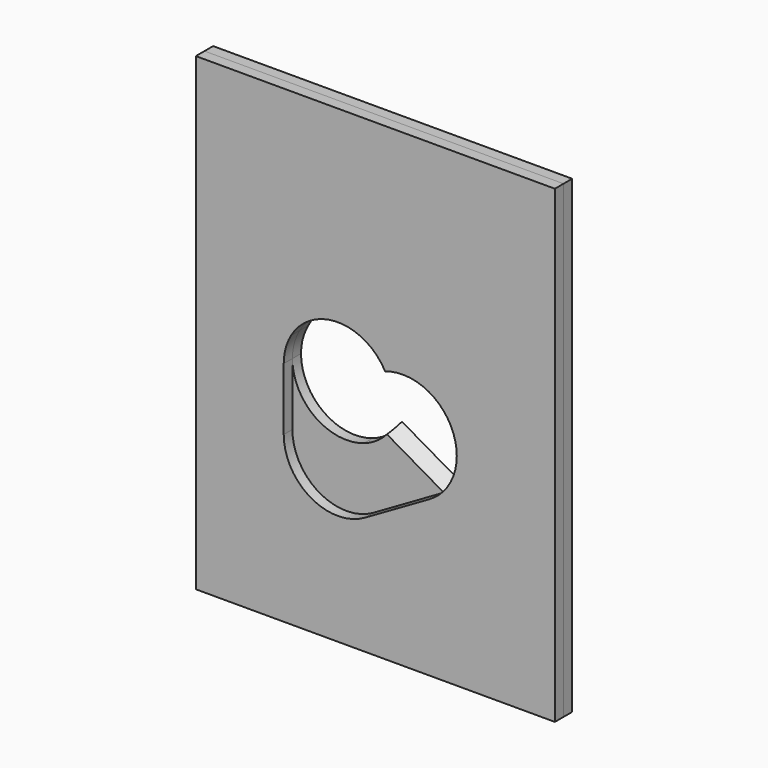
from build123d import *

# Parameters (mm, degrees)
F0_W     = 332.0041149855
F0_H     = 434.023141861
F1_DEPTH = 10
F2_DEPTH = 10
F3_SIZE  = 9.99999


# Not quite as in the source:
# - a fillet or chamfer is up to 0.001 mm smaller than in the source, because OpenCascade refuses the exact size


with BuildPart() as f1:
    # F0 (on Front) → F1 (new body)
    with BuildSketch(Plane.XZ):
        with Locations((34.709520638, 6.8919658661)):
            Rectangle(F0_W, F0_H)
        with BuildLine():
            ThreePointArc((-50, 0), (-48.2962913145, 12.9409522551), (-43.3012701892, 25))
            Line((-43.3012701892, 25), (16.6987298108, 128.9230484541))
            ThreePointArc((16.6987298108, 128.9230484541), (72.9409522551, 152.2193397686), (110, 103.9230484541))
            Line((110, 103.9230484541), (110, -23.0940107676))
            Line((110, -23.0940107676), (110, -63.5085296109))
            Line((110, -63.5085296109), (97.4264068712, -56.2491622333))
            ThreePointArc((97.4264068712, -56.2491622333), (91.6227766017, -61.8238442297), (85, -66.3952809568))
            Line((85, -66.3952809568), (50, -86.6025403784))
            Line((50, -86.6025403784), (25, -101.0362971082))
            ThreePointArc((25, -101.0362971082), (-25, -101.0362971082), (-50, -57.735026919))
            Line((-50, -57.735026919), (-50, 0))
        make_face(mode=Mode.SUBTRACT)
        with BuildLine():
            ThreePointArc((-40.8248290464, -28.8675134595), (-47.6510306936, -15.1452723264), (-50, 0))
            Line((-50, 0), (-50, -57.735026919))
            ThreePointArc((-50, -57.735026919), (-47.6510306936, -42.5897545926), (-40.8248290464, -28.8675134595))
        make_face()
        with BuildLine():
            ThreePointArc((16.2432812114, -47.2880092147), (-15.3587691387, -47.582646107), (-40.8248290464, -28.8675134595))
            ThreePointArc((-40.8248290464, -28.8675134595), (-47.6510306936, -42.5897545926), (-50, -57.735026919))
            ThreePointArc((-50, -57.735026919), (-25, -101.0362971082), (25, -101.0362971082))
            ThreePointArc((25, -101.0362971082), (36.9417059287, -91.4293938529), (45.4124145232, -78.6566092486))
            Line((45.4124145232, -78.6566092486), (39.7196014439, -68.7963677572))
            ThreePointArc((39.7196014439, -68.7963677572), (26.2236699558, -59.9607915973), (16.2432812114, -47.2880092147))
        make_face()
        with BuildLine():
            ThreePointArc((25, -43.3012701892), (20.7177600933, -45.5057624561), (16.2432812114, -47.2880092147))
            ThreePointArc((16.2432812114, -47.2880092147), (26.2236699558, -59.9607915973), (39.7196014439, -68.7963677572))
            Line((39.7196014439, -68.7963677572), (25, -43.3012701892))
        make_face()
        with BuildLine():
            ThreePointArc((48.0277563773, -71.6395088353), (43.8111428854, -70.400679487), (39.7196014439, -68.7963677572))
            Line((39.7196014439, -68.7963677572), (45.4124145232, -78.6566092486))
            ThreePointArc((45.4124145232, -78.6566092486), (46.8516414764, -75.1970912576), (48.0277563773, -71.6395088353))
        make_face()
        with BuildLine():
            ThreePointArc((50, -57.735026919), (47.6510306936, -42.5897545926), (40.8248290464, -28.8675134595))
            ThreePointArc((40.8248290464, -28.8675134595), (33.694366934, -36.9417059287), (25, -43.3012701892))
            Line((25, -43.3012701892), (39.7196014439, -68.7963677572))
            ThreePointArc((39.7196014439, -68.7963677572), (43.8111428854, -70.400679487), (48.0277563773, -71.6395088353))
            ThreePointArc((48.0277563773, -71.6395088353), (49.5044837306, -64.756856493), (50, -57.735026919))
        make_face()
        with BuildLine():
            Line((97.4264068712, -56.2491622333), (43.3012701892, -25))
            ThreePointArc((43.3012701892, -25), (42.1074762749, -26.9622039485), (40.8248290464, -28.8675134595))
            ThreePointArc((40.8248290464, -28.8675134595), (47.6510306936, -42.5897545926), (50, -57.735026919))
            ThreePointArc((50, -57.735026919), (49.5044837306, -64.756856493), (48.0277563773, -71.6395088353))
            ThreePointArc((48.0277563773, -71.6395088353), (67.021829574, -72.5984944982), (85, -66.3952809568))
            ThreePointArc((85, -66.3952809568), (91.6227766017, -61.8238442297), (97.4264068712, -56.2491622333))
        make_face()
        with BuildLine():
            Line((50, -86.6025403784), (85, -66.3952809568))
            ThreePointArc((85, -66.3952809568), (67.021829574, -72.5984944982), (48.0277563773, -71.6395088353))
            ThreePointArc((48.0277563773, -71.6395088353), (46.8516414764, -75.1970912576), (45.4124145232, -78.6566092486))
            Line((45.4124145232, -78.6566092486), (50, -86.6025403784))
        make_face()
        with BuildLine():
            ThreePointArc((45.4124145232, -78.6566092486), (36.9417059287, -91.4293938529), (25, -101.0362971082))
            Line((25, -101.0362971082), (50, -86.6025403784))
            Line((50, -86.6025403784), (45.4124145232, -78.6566092486))
        make_face()
    extrude(amount=-F1_DEPTH)

    # F3 (size 10 in the source; OpenCascade refuses exactly that, so slightly less here)
    f3_edges = [f1.edges().sort_by_distance(p)[0] for p in [
        (76.650635, 0, -44.254265),
    ]]
    chamfer(f3_edges, length=F3_SIZE)


with BuildPart() as f2:
    # F0 (on Front) → F2 (new body)
    with BuildSketch(Plane.XZ):
        with Locations((34.709520638, 6.8919658661)):
            Rectangle(F0_W, F0_H)
        with BuildLine():
            ThreePointArc((-50, 0), (-48.2962913145, 12.9409522551), (-43.3012701892, 25))
            Line((-43.3012701892, 25), (16.6987298108, 128.9230484541))
            ThreePointArc((16.6987298108, 128.9230484541), (72.9409522551, 152.2193397686), (110, 103.9230484541))
            Line((110, 103.9230484541), (110, -23.0940107676))
            Line((110, -23.0940107676), (110, -63.5085296109))
            Line((110, -63.5085296109), (97.4264068712, -56.2491622333))
            ThreePointArc((97.4264068712, -56.2491622333), (91.6227766017, -61.8238442297), (85, -66.3952809568))
            Line((85, -66.3952809568), (50, -86.6025403784))
            Line((50, -86.6025403784), (25, -101.0362971082))
            ThreePointArc((25, -101.0362971082), (-25, -101.0362971082), (-50, -57.735026919))
            Line((-50, -57.735026919), (-50, 0))
        make_face(mode=Mode.SUBTRACT)
        with BuildLine():
            ThreePointArc((110, 103.9230484541), (72.9409522551, 152.2193397686), (16.6987298108, 128.9230484541))
            ThreePointArc((16.6987298108, 128.9230484541), (47.0590477449, 55.6267571397), (110, 103.9230484541))
        make_face()
        with BuildLine():
            ThreePointArc((-43.3012701892, 25), (0, 50), (43.3012701892, 25))
            ThreePointArc((43.3012701892, 25), (43.5308599828, 24.5980533612), (43.7567187886, 24.1939984471))
            ThreePointArc((43.7567187886, 24.1939984471), (89.0502662589, 17.6009770108), (110, -23.0940107676))
            Line((110, -23.0940107676), (110, 103.9230484541))
            ThreePointArc((110, 103.9230484541), (47.0590477449, 55.6267571397), (16.6987298108, 128.9230484541))
            Line((16.6987298108, 128.9230484541), (-43.3012701892, 25))
        make_face()
        with BuildLine():
            Line((110, -63.5085296109), (110, -23.0940107676))
            ThreePointArc((110, -23.0940107676), (106.7510446063, -40.8236421292), (97.4264068712, -56.2491622333))
            Line((97.4264068712, -56.2491622333), (110, -63.5085296109))
        make_face()
    extrude(amount=F2_DEPTH)


solid = Compound([f1.part, f2.part])
